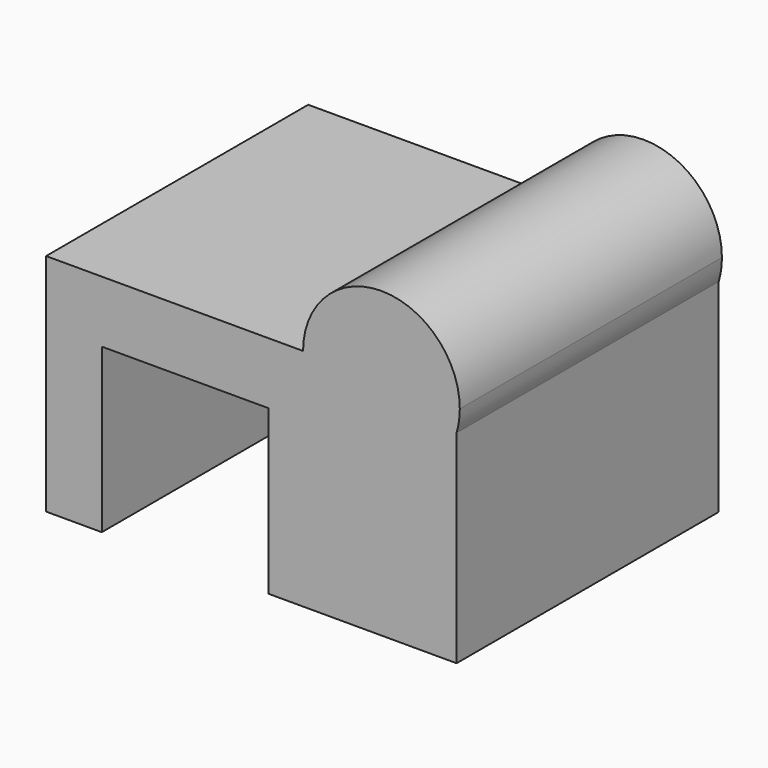
from build123d import *

# Parameters (mm, degrees)
F1_DEPTH = 25.4
F2_W     = 12.9091180861
F2_H     = 25.0910650939
F3_DEPTH = 28.702


with BuildPart() as f1:
    # F0 (on Front) → F1 (new body)
    with BuildSketch(Plane.XZ):
        with BuildLine():
            Line((-33.6216918521, 56.1617612839), (-53.54340747, 56.1617612839))
            Line((-53.54340747, 56.1617612839), (-53.54340747, 38.7188270688))
            Line((-53.54340747, 38.7188270688), (-21.719571203, 38.7188270688))
            Line((-21.719571203, 38.7188270688), (-21.719571203, 54.4453912809))
            ThreePointArc((-21.719571203, 54.4453912809), (-28.4139375356, 50.1491411825), (-33.6216918521, 56.1617612839))
        make_face()
        with BuildLine():
            ThreePointArc((-21.4720585056, 56.1617612839), (-27.5468751788, 62.2365779571), (-33.6216918521, 56.1617612839))
            Line((-33.6216918521, 56.1617612839), (-21.719571203, 56.1617612839))
            Line((-21.719571203, 56.1617612839), (-21.719571203, 54.4453912809))
            ThreePointArc((-21.719571203, 54.4453912809), (-21.5342550775, 55.2946989271), (-21.4720585056, 56.1617612839))
        make_face()
        with BuildLine():
            Line((-21.719571203, 56.1617612839), (-33.6216918521, 56.1617612839))
            ThreePointArc((-33.6216918521, 56.1617612839), (-28.4139375356, 50.1491411825), (-21.719571203, 54.4453912809))
            Line((-21.719571203, 54.4453912809), (-21.719571203, 56.1617612839))
        make_face()
    extrude(amount=F1_DEPTH)

    # F2 (on Front) → F3 (cut)
    with BuildSketch(Plane.XZ):
        with Locations((-42.769966647, 38.8393672183)):
            Rectangle(F2_W, F2_H)
    extrude(amount=F3_DEPTH, mode=Mode.SUBTRACT)


solid = f1.part
